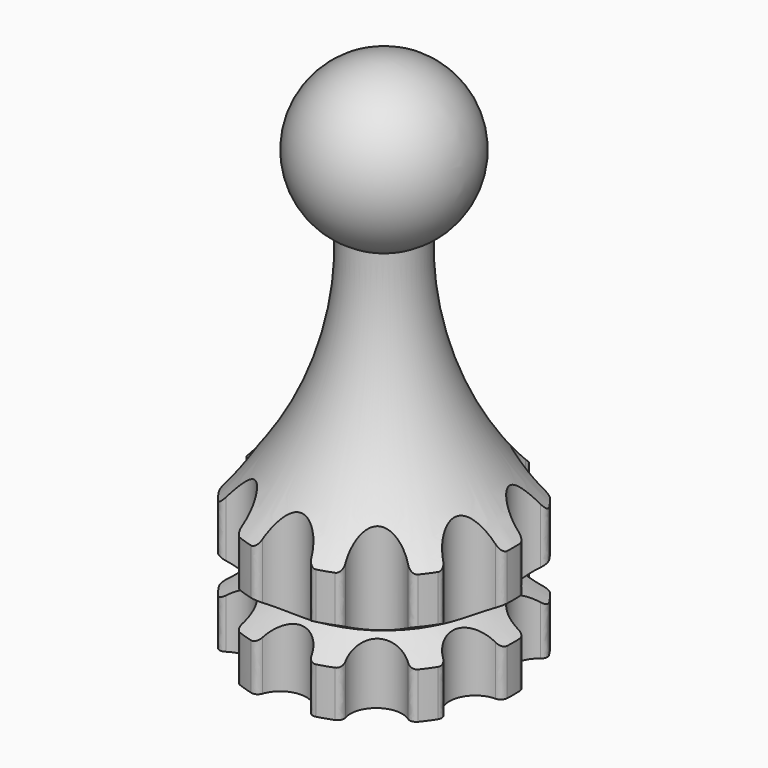
from build123d import *

# Parameters (mm, degrees)
F2_R            = 4
F3_DEPTH        = 30
F3_COPIES_COUNT = 10
F4_R            = 1


# Not quite as in the source:
# - a pattern or mirror of a feature is missing from the dataset's text; its kind, count and spacing are read off the source's solid


with BuildPart() as f1:
    # F0 (on Front) → F1 (revolve)
    with BuildSketch(Plane.XZ):
        with BuildLine():
            Line((0, 0), (20, 0))
            Line((20, 0), (20, 7.1132486541))
            Line((20, 7.1132486541), (15, 10))
            Line((15, 10), (20, 12.8867513459))
            Line((20, 12.8867513459), (20, 20))
            ThreePointArc((20, 20), (9.2781887481, 36.8408620554), (6, 56.5341439003))
            ThreePointArc((6, 56.5341439003), (12.1103922572, 70.5965140685), (0, 80))
            Line((0, 80), (0, 0))
        make_face()
    revolve(axis=Axis((0, 0, 40), (0, 0, -1)))

    # F2 (on face) → F3 (cut)
    with BuildSketch(Plane(origin=(0, 0, 0), x_dir=(1, 0, 0), z_dir=(0, 0, -1))):
        with Locations((0, 20)):
            Circle(F2_R)
    f3 = extrude(amount=-F3_DEPTH, mode=Mode.SUBTRACT)

    # F3_copies: F3 ×10 about axis
    f3_copies_axis = Axis((0, 0, 0), (0, 0, 1))
    for i in range(1, F3_COPIES_COUNT):
        add(f3.rotate(f3_copies_axis, i * 360 / F3_COPIES_COUNT), mode=Mode.SUBTRACT)

    # F4
    f4_edges = [f1.edges().sort_by_distance(p)[0] for p in [
        (3.97995, -19.6, 16.443376),
        (-3.97995, -19.6, 16.443376),
        (3.97995, -19.6, 3.556624),
        (-3.97995, -19.6, 3.556624),
        (19.87058, 2.271576, 16.443376),
        (19.87058, -2.271576, 16.443376),
        (17.410836, 9.84189, 16.443376),
        (14.740438, 13.517377, 16.443376),
        (8.300744, 18.196089, 16.443376),
        (3.97995, 19.6, 16.443376),
        (-3.97995, 19.6, 16.443376),
        (-8.300744, 18.196089, 16.443376),
        (-14.740438, 13.517377, 16.443376),
        (-17.410836, 9.84189, 16.443376),
        (-19.87058, 2.271576, 16.443376),
        (-19.87058, -2.271576, 16.443376),
        (-17.410836, -9.84189, 16.443376),
        (-14.740438, -13.517377, 16.443376),
        (-8.300744, -18.196089, 16.443376),
        (8.300744, -18.196089, 16.443376),
        (14.740438, -13.517377, 16.443376),
        (17.410836, -9.84189, 16.443376),
        (8.300744, -18.196089, 3.556624),
        (14.740438, -13.517377, 3.556624),
        (17.410836, -9.84189, 3.556624),
        (19.87058, -2.271576, 3.556624),
        (19.87058, 2.271576, 3.556624),
        (17.410836, 9.84189, 3.556624),
        (14.740438, 13.517377, 3.556624),
        (8.300744, 18.196089, 3.556624),
        (3.97995, 19.6, 3.556624),
        (-3.97995, 19.6, 3.556624),
        (-8.300744, 18.196089, 3.556624),
        (-14.740438, 13.517377, 3.556624),
        (-17.410836, 9.84189, 3.556624),
        (-19.87058, 2.271576, 3.556624),
        (-19.87058, -2.271576, 3.556624),
        (-17.410836, -9.84189, 3.556624),
        (-14.740438, -13.517377, 3.556624),
        (-8.300744, -18.196089, 3.556624),
    ]]
    fillet(f4_edges, radius=F4_R)


solid = f1.part
